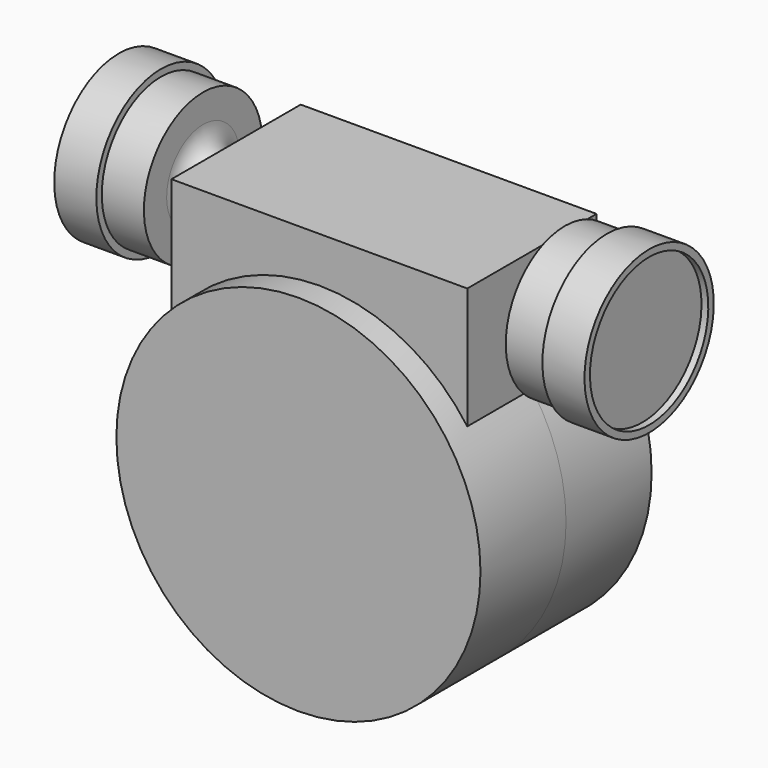
from build123d import *

# Parameters (mm, degrees)
F0_R      = 80
F1_DEPTH  = 47
F2_W      = 130
F2_H      = 71
F3_DEPTH  = 100
F4_W      = 79.5
F4_H      = 10
F6_R      = 10
F7_R      = 80
F8_DEPTH  = 47
F9_R      = 55
F10_DEPTH = 3


# Not quite as in the source:
# - a pattern or mirror of a feature is missing from the dataset's text; its kind, count and spacing are read off the source's solid


with BuildPart() as f1:
    # F0 (on Front) → F1 (new body)
    with BuildSketch(Plane.XZ):
        Circle(F0_R)
    extrude(amount=F1_DEPTH)

    # F2 (on Top) → F3 (join)
    with BuildSketch(Plane.XY):
        Rectangle(F2_W, F2_H)
    extrude(amount=F3_DEPTH)

    # F4 (on Front) → F5 (revolve)
    with BuildSketch(Plane.XZ):
        Polygon((79.5, 114.5), (79.5, 92), (79.5, 82), (113.5, 82), (113.5, 114.5), (116.5, 114.5), (116.5, 117.5), (98, 117.5), (98, 114.5), align=None)
        with Locations((39.75, 87)):
            Rectangle(F4_W, F4_H)
    f5 = revolve(axis=Axis((96.5, 0, 82), (-1, 0, 0)))

    # F5_copies: F5 across plane
    add(f5.mirror(Plane(origin=(0, 0, 0), x_dir=(0, 0, -1), z_dir=(-1, 0, 0))))

    # F6
    f6_edges = [f1.edges().sort_by_distance(p)[0] for p in [
        (79.5, 0, 72),
        (-79.5, 0, 72),
    ]]
    fillet(f6_edges, radius=F6_R)

    # F7 (on Front) → F8 (join)
    with BuildSketch(Plane.XZ):
        Circle(F7_R)
    extrude(amount=-F8_DEPTH)

    # F9 (on face) → F10 (cut)
    with BuildSketch(Plane(origin=(0, 47, 0), x_dir=(-1, 0, 0), z_dir=(0, 1, 0))):
        Circle(F9_R)
    extrude(amount=-F10_DEPTH, mode=Mode.SUBTRACT)


solid = f1.part
